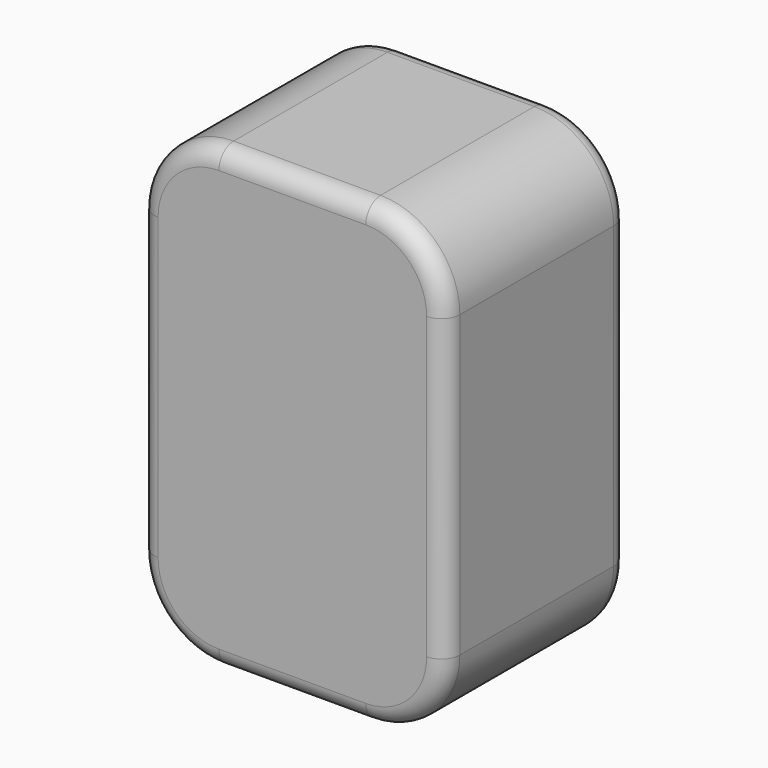
from build123d import *

# Parameters (mm, degrees)
F0_W         = 101.6
F0_H         = 76.2
F1_DEPTH     = 152.4
F2_W         = 76.2
F2_H         = 25.4
F3_DEPTH     = 50.8
F4_R         = 26.3680405282
F5_T1_DEPTH  = 48.8639189435
F5_T3_DEPTH  = 99.6639189435
F5_T6_ANGLE  = 90
F5_T8_ANGLE  = 90
F5_T10_ANGLE = 90
F5_T12_ANGLE = 90
F5_T14_ANGLE = 90
F5_T16_ANGLE = 90
F5_T18_ANGLE = 90
F5_T20_ANGLE = 90


# Not quite as in the source:
# - a fillet or chamfer that OpenCascade refuses, or shapes differently, is made with other operations: its cross-section is extruded or revolved along the edge and cut away or added


with BuildPart() as f1:
    # F0 (on Top) → F1 (new body)
    with BuildSketch(Plane.XY):
        with Locations((-0.5902759731, -8.3016921655)):
            Rectangle(F0_W, F0_H)
    extrude(amount=F1_DEPTH)

    # F2 (on face) → F3 (cut)
    with BuildSketch(Plane(origin=(0, 29.7983078345, 0), x_dir=(-1, 0, 0), z_dir=(0, 1, 0))):
        with Locations((0.5902759731, 129.54)):
            Rectangle(F2_W, F2_H)
        with Locations((0.5074083115, 93.9800965559)):
            Rectangle(F2_W, F2_H)
        with Locations((0.42454065, 58.4201931119)):
            Rectangle(F2_W, F2_H)
        with Locations((0.3416729884, 22.8602896678)):
            Rectangle(F2_W, F2_H)
    extrude(amount=-F3_DEPTH, mode=Mode.SUBTRACT)

    # F4
    f4_edges = [f1.edges().sort_by_distance(p)[0] for p in [
        (-51.390276, -8.301692, 152.4),
        (50.209724, -8.301692, 152.4),
        (-51.390276, -8.301692, 0),
        (50.209724, -8.301692, 0),
    ]]
    fillet(f4_edges, radius=F4_R)

    # F5: fillet of radius 6.1321024484 on 16 edges, made by hand

    # F5_s2 → F5_t1 (cut)
    with BuildSketch(Plane.YZ.offset(-25.0222354448)):
        with BuildLine():
            ThreePointArc((23.6662053861, 152.4), (28.0022566103, 150.6039487758), (29.7983078345, 146.2678975516))
            Line((29.7983078345, 146.2678975516), (29.7983078345, 152.4))
            Line((29.7983078345, 152.4), (23.6662053861, 152.4))
        make_face()
        with BuildLine():
            ThreePointArc((-46.4016921655, 146.2678975516), (-44.6056409413, 150.6039487758), (-40.2695897171, 152.4))
            Line((-40.2695897171, 152.4), (-46.4016921655, 152.4))
            Line((-46.4016921655, 152.4), (-46.4016921655, 146.2678975516))
        make_face()
        with BuildLine():
            ThreePointArc((23.6662053861, 0), (28.0022566103, 1.7960512242), (29.7983078345, 6.1321024484))
            Line((29.7983078345, 6.1321024484), (29.7983078345, 0))
            Line((29.7983078345, 0), (23.6662053861, 0))
        make_face()
        with BuildLine():
            ThreePointArc((-46.4016921655, 6.1321024484), (-44.6056409413, 1.7960512242), (-40.2695897171, 0))
            Line((-40.2695897171, 0), (-46.4016921655, 0))
            Line((-46.4016921655, 0), (-46.4016921655, 6.1321024484))
        make_face()
    extrude(amount=F5_T1_DEPTH, mode=Mode.SUBTRACT)

    # F5_s4 → F5_t3 (cut)
    with BuildSketch(Plane.XY.offset(26.3680405282)):
        with BuildLine():
            ThreePointArc((-45.2581735247, -46.4016921655), (-49.5942247489, -44.6056409413), (-51.3902759731, -40.2695897171))
            Line((-51.3902759731, -40.2695897171), (-51.3902759731, -46.4016921655))
            Line((-51.3902759731, -46.4016921655), (-45.2581735247, -46.4016921655))
        make_face()
        with BuildLine():
            ThreePointArc((44.0776215785, -46.4016921655), (48.4136728027, -44.6056409413), (50.2097240269, -40.2695897171))
            Line((50.2097240269, -40.2695897171), (50.2097240269, -46.4016921655))
            Line((50.2097240269, -46.4016921655), (44.0776215785, -46.4016921655))
        make_face()
        with BuildLine():
            ThreePointArc((-51.3902759731, 23.6662053861), (-49.5942247489, 28.0022566103), (-45.2581735247, 29.7983078345))
            Line((-45.2581735247, 29.7983078345), (-51.3902759731, 29.7983078345))
            Line((-51.3902759731, 29.7983078345), (-51.3902759731, 23.6662053861))
        make_face()
        with BuildLine():
            ThreePointArc((50.2097240269, 23.6662053861), (48.4136728027, 28.0022566103), (44.0776215785, 29.7983078345))
            Line((44.0776215785, 29.7983078345), (50.2097240269, 29.7983078345))
            Line((50.2097240269, 29.7983078345), (50.2097240269, 23.6662053861))
        make_face()
    extrude(amount=F5_T3_DEPTH, mode=Mode.SUBTRACT)

    # F5_s5 → F5_t6 (revolve, cut)
    with BuildSketch(Plane.XY.offset(26.3680405282)):
        with BuildLine():
            ThreePointArc((-45.2581735247, -46.4016921655), (-49.5942247489, -44.6056409413), (-51.3902759731, -40.2695897171))
            Line((-51.3902759731, -40.2695897171), (-51.3902759731, -46.4016921655))
            Line((-51.3902759731, -46.4016921655), (-45.2581735247, -46.4016921655))
        make_face()
    revolve(axis=Axis((-25.0222354448, -46.4016921655, 26.3680405282), (0, -1, 0)), revolution_arc=F5_T6_ANGLE, mode=Mode.SUBTRACT)

    # F5_s7 → F5_t8 (revolve, cut)
    with BuildSketch(Plane.XY.offset(126.0319594718)):
        with BuildLine():
            ThreePointArc((-45.2581735247, -46.4016921655), (-49.5942247489, -44.6056409413), (-51.3902759731, -40.2695897171))
            Line((-51.3902759731, -40.2695897171), (-51.3902759731, -46.4016921655))
            Line((-51.3902759731, -46.4016921655), (-45.2581735247, -46.4016921655))
        make_face()
    revolve(axis=Axis((-25.0222354448, -46.4016921655, 126.0319594718), (0, 1, 0)), revolution_arc=F5_T8_ANGLE, mode=Mode.SUBTRACT)

    # F5_s9 → F5_t10 (revolve, cut)
    with BuildSketch(Plane.XY.offset(26.3680405282)):
        with BuildLine():
            ThreePointArc((44.0776215785, -46.4016921655), (48.4136728027, -44.6056409413), (50.2097240269, -40.2695897171))
            Line((50.2097240269, -40.2695897171), (50.2097240269, -46.4016921655))
            Line((50.2097240269, -46.4016921655), (44.0776215785, -46.4016921655))
        make_face()
    revolve(axis=Axis((23.8416834987, -46.4016921655, 26.3680405282), (0, 1, 0)), revolution_arc=F5_T10_ANGLE, mode=Mode.SUBTRACT)

    # F5_s11 → F5_t12 (revolve, cut)
    with BuildSketch(Plane.XY.offset(126.0319594718)):
        with BuildLine():
            ThreePointArc((44.0776215785, -46.4016921655), (48.4136728027, -44.6056409413), (50.2097240269, -40.2695897171))
            Line((50.2097240269, -40.2695897171), (50.2097240269, -46.4016921655))
            Line((50.2097240269, -46.4016921655), (44.0776215785, -46.4016921655))
        make_face()
    revolve(axis=Axis((23.8416834987, -46.4016921655, 126.0319594718), (0, -1, 0)), revolution_arc=F5_T12_ANGLE, mode=Mode.SUBTRACT)

    # F5_s13 → F5_t14 (revolve, cut)
    with BuildSketch(Plane.XY.offset(26.3680405282)):
        with BuildLine():
            ThreePointArc((-51.3902759731, 23.6662053861), (-49.5942247489, 28.0022566103), (-45.2581735247, 29.7983078345))
            Line((-45.2581735247, 29.7983078345), (-51.3902759731, 29.7983078345))
            Line((-51.3902759731, 29.7983078345), (-51.3902759731, 23.6662053861))
        make_face()
    revolve(axis=Axis((-25.0222354448, 29.7983078345, 26.3680405282), (0, -1, 0)), revolution_arc=F5_T14_ANGLE, mode=Mode.SUBTRACT)

    # F5_s15 → F5_t16 (revolve, cut)
    with BuildSketch(Plane.XY.offset(126.0319594718)):
        with BuildLine():
            ThreePointArc((-51.3902759731, 23.6662053861), (-49.5942247489, 28.0022566103), (-45.2581735247, 29.7983078345))
            Line((-45.2581735247, 29.7983078345), (-51.3902759731, 29.7983078345))
            Line((-51.3902759731, 29.7983078345), (-51.3902759731, 23.6662053861))
        make_face()
    revolve(axis=Axis((-25.0222354448, 29.7983078345, 126.0319594718), (0, 1, 0)), revolution_arc=F5_T16_ANGLE, mode=Mode.SUBTRACT)

    # F5_s17 → F5_t18 (revolve, cut)
    with BuildSketch(Plane.XY.offset(26.3680405282)):
        with BuildLine():
            ThreePointArc((50.2097240269, 23.6662053861), (48.4136728027, 28.0022566103), (44.0776215785, 29.7983078345))
            Line((44.0776215785, 29.7983078345), (50.2097240269, 29.7983078345))
            Line((50.2097240269, 29.7983078345), (50.2097240269, 23.6662053861))
        make_face()
    revolve(axis=Axis((23.8416834987, 29.7983078345, 26.3680405282), (0, 1, 0)), revolution_arc=F5_T18_ANGLE, mode=Mode.SUBTRACT)

    # F5_s19 → F5_t20 (revolve, cut)
    with BuildSketch(Plane.XY.offset(126.0319594718)):
        with BuildLine():
            ThreePointArc((50.2097240269, 23.6662053861), (48.4136728027, 28.0022566103), (44.0776215785, 29.7983078345))
            Line((44.0776215785, 29.7983078345), (50.2097240269, 29.7983078345))
            Line((50.2097240269, 29.7983078345), (50.2097240269, 23.6662053861))
        make_face()
    revolve(axis=Axis((23.8416834987, 29.7983078345, 126.0319594718), (0, -1, 0)), revolution_arc=F5_T20_ANGLE, mode=Mode.SUBTRACT)


solid = f1.part
